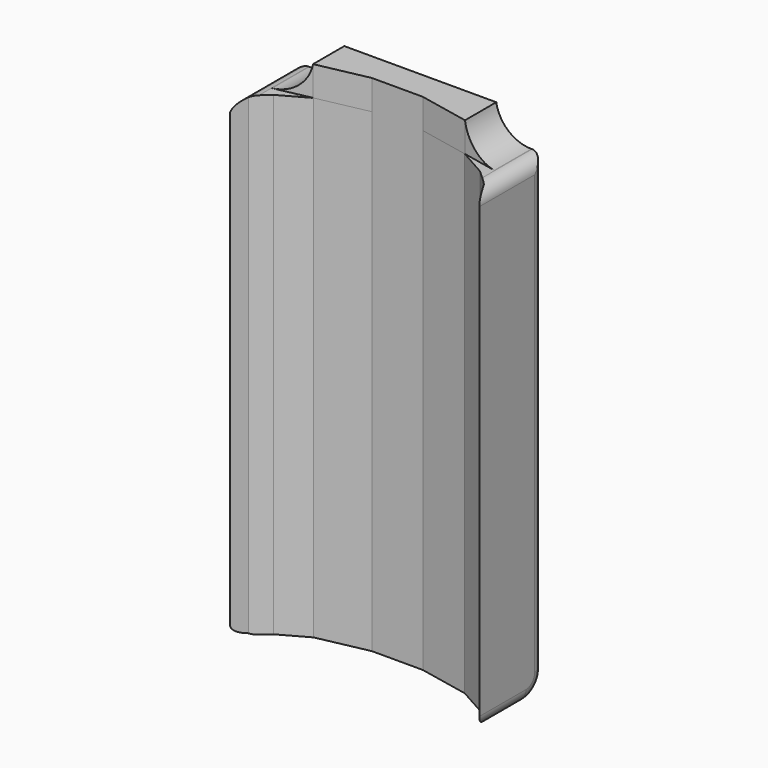
from build123d import *

# Parameters (mm, degrees)
F1_DEPTH    = 50.8
F4_DEPTH    = 3.175
F5_T4_DEPTH = 13.5737083661
F5_T9_DEPTH = 13.5737083661
F6_R        = 1.397
F7_T1_DEPTH = 26.6857916153
F7_T4_ANGLE = 90
F7_T6_ANGLE = 90


# Not quite as in the source:
# - a fillet or chamfer that OpenCascade refuses, or shapes differently, is made with other operations: its cross-section is extruded or revolved along the edge and cut away or added


with BuildPart() as f1:
    # F0 (on Top) → F1 (new body)
    with BuildSketch(Plane.XY):
        Polygon((16.83116441, 6.3822651147), (-9.8546272053, 6.3822651147), (-9.8546272053, -2.4114359531), (-9.1195573698, -0.8609411879), (-7.5529336119, 0.5598957894), (-4.6044890144, 2.2076013963), (0.7639104889, 3.3147196292), (6.2126267158, 3.3147196292), (11.5810262191, 2.2076013963), (14.5294708166, 0.5598957894), (16.0960945745, -0.8609411879), (16.83116441, -2.4114359531), align=None)
    extrude(amount=F1_DEPTH)

    # F3 (on face) → F4 (join)
    with BuildSketch(Plane.XY.offset(50.8)):
        Polygon((11.6162686024, 6.3822651147), (-4.6397313976, 6.3822651147), (-4.6397313976, 2.2003334042), (0.7639104889, 3.3147196292), (6.2126267158, 3.3147196292), (11.6162686024, 2.2003334042), align=None)
    extrude(amount=F4_DEPTH)

    # F5: fillet of radius 3.81 on 2 edges, made by hand


with BuildPart() as f5_tool2:
    # F5_s3 → F5_t4 (new body)
    with BuildSketch(Plane.XZ.offset(7.1914432514)):
        with BuildLine():
            ThreePointArc((15.3729792646, 50.8), (12.9136348398, 51.7000644337), (11.6162686024, 53.975))
            Line((11.6162686024, 53.975), (11.6162686024, 50.8))
            Line((11.6162686024, 50.8), (15.3729792646, 50.8))
        make_face()
    extrude(amount=-F5_T4_DEPTH)

    split(bisect_by=Plane(origin=(0.9091488864, 4.4084491475, 0), x_dir=(0, 0, 1), z_dir=(0.2019783567, 0.9793899854, 0)), keep=Keep.TOP)


with BuildPart() as f1_1:
    add(f1.part)

    # F5_t1: union F5_tool2
    add(f5_tool2.part)


with BuildPart() as f5_tool7:
    # F5_s8 → F5_t9 (new body)
    with BuildSketch(Plane.XZ.offset(-6.3822651147)):
        with BuildLine():
            ThreePointArc((-8.3964420599, 50.8), (-5.9370976351, 51.7000644337), (-4.6397313976, 53.975))
            Line((-4.6397313976, 53.975), (-4.6397313976, 50.8))
            Line((-4.6397313976, 50.8), (-8.3964420599, 50.8))
        make_face()
    extrude(amount=F5_T9_DEPTH)

    split(bisect_by=Plane(origin=(-0.624539261, 3.0283813951, 0), x_dir=(0, 0, 1), z_dir=(-0.2019783567, 0.9793899854, 0)), keep=Keep.TOP)


with BuildPart() as f1_2:
    add(f1_1.part)

    # F5_t6: union F5_tool7
    add(f5_tool7.part)

    # F6
    f6_edges = [f1_2.edges().sort_by_distance(p)[0] for p in [
        (-9.854627, 1.985415, 50.8),
        (16.831164, 1.985415, 50.8),
        (16.831164, 1.985415, 0),
        (-9.854627, 1.985415, 0),
        (16.831164, 6.382265, 25.4),
        (-9.854627, 6.382265, 25.4),
    ]]
    fillet(f6_edges, radius=F6_R)

    # F7: fillet of radius 2.54 on 1 edges, made by hand

    # F7_s2 → F7_t1 (cut)
    with BuildSketch(Plane.YZ.offset(-9.8546272053)):
        with BuildLine():
            ThreePointArc((6.3822651147, 2.54), (5.6383163389, 0.7439487758), (3.8422651147, 0))
            Line((3.8422651147, 0), (6.3822651147, 0))
            Line((6.3822651147, 0), (6.3822651147, 2.54))
        make_face()
    extrude(amount=F7_T1_DEPTH, mode=Mode.SUBTRACT)

    # F7_s3 → F7_t4 (revolve, cut)
    with BuildSketch(Plane.XZ.offset(-3.8422651147)):
        with BuildLine():
            ThreePointArc((16.83116441, 1.397), (16.4219925833, 0.4091718267), (15.43416441, 0))
            Line((15.43416441, 0), (16.83116441, 0))
            Line((16.83116441, 0), (16.83116441, 1.397))
        make_face()
    revolve(axis=Axis((16.83116441, 3.8422651147, 2.54), (1, 0, 0)), revolution_arc=F7_T4_ANGLE, mode=Mode.SUBTRACT)

    # F7_s5 → F7_t6 (revolve, cut)
    with BuildSketch(Plane.XY.offset(2.54)):
        with BuildLine():
            ThreePointArc((-9.8546272053, 4.9852651147), (-9.4454553786, 5.973093288), (-8.4576272053, 6.3822651147))
            Line((-8.4576272053, 6.3822651147), (-9.8546272053, 6.3822651147))
            Line((-9.8546272053, 6.3822651147), (-9.8546272053, 4.9852651147))
        make_face()
    revolve(axis=Axis((-9.8546272053, 3.8422651147, 2.54), (-1, 0, 0)), revolution_arc=F7_T6_ANGLE, mode=Mode.SUBTRACT)


solid = f1_2.part
